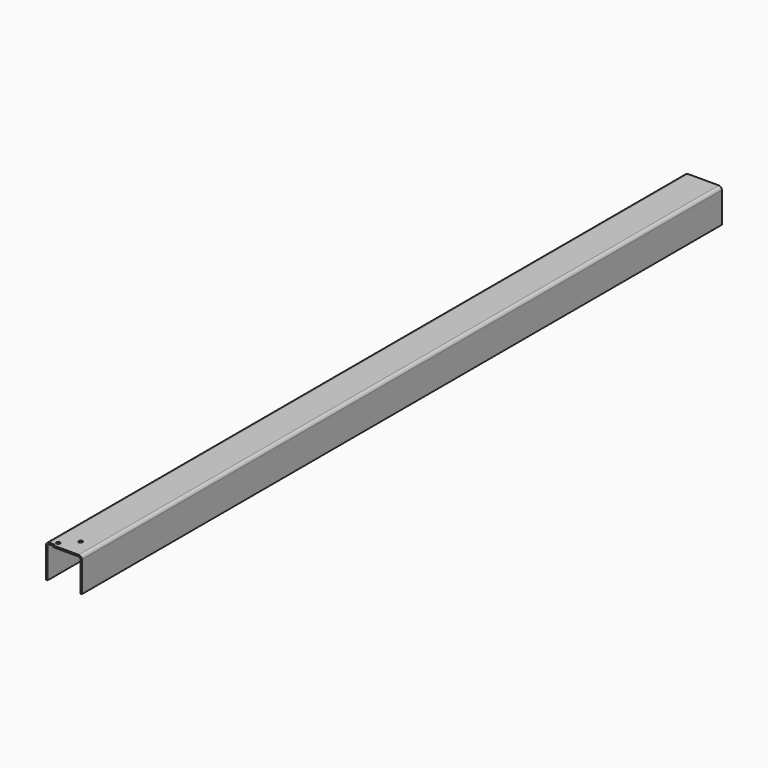
from build123d import *

# Parameters (mm, degrees)
F1_DEPTH = 1996
F3_W     = 4
F3_H     = 87
F4_DEPTH = 21.409
F6_DEPTH = 4.001


with BuildPart() as f1:
    # F0 (on Front) → F1 (new body)
    with BuildSketch(Plane.XZ):
        with BuildLine():
            Line((-46.25, 34), (-46.25, -42))
            Line((-46.25, -42), (-42.25, -42))
            Line((-42.25, -42), (-42.25, 34))
            ThreePointArc((-42.25, 34), (-41.0784271247, 36.8284271247), (-38.25, 38))
            Line((-38.25, 38), (38.25, 38))
            ThreePointArc((38.25, 38), (41.0784271247, 36.8284271247), (42.25, 34))
            Line((42.25, 34), (42.25, -42))
            Line((42.25, -42), (46.25, -42))
            Line((46.25, -42), (46.25, 34))
            ThreePointArc((46.25, 34), (43.9068542495, 39.6568542495), (38.25, 42))
            Line((38.25, 42), (-38.25, 42))
            ThreePointArc((-38.25, 42), (-43.9068542495, 39.6568542495), (-46.25, 34))
        make_face()
    extrude(amount=-F1_DEPTH)

    # F3 (on face) → F4 (cut)
    with BuildSketch(Plane(origin=(-46.25, 0, 0), x_dir=(0, -1, 0), z_dir=(-1, 0, 0))):
        with Locations((-2, 0.3707238951)):
            Rectangle(F3_W, F3_H)
    extrude(amount=-F4_DEPTH, mode=Mode.SUBTRACT)

    # F5 (on face) → F6 (cut, through all)
    with BuildSketch(Plane(origin=(0, 0, 38), x_dir=(1, 0, 0), z_dir=(0, 0, -1))):
        with BuildLine():
            ThreePointArc((-19.7495876579, -14.5), (-21.0676071426, -11.3180194847), (-24.2495876579, -10))
            ThreePointArc((-24.2495876579, -10), (-28.7495876579, -14.5), (-24.2495876579, -19))
            ThreePointArc((-24.2495876579, -19), (-21.0676071426, -17.6819805153), (-19.7495876579, -14.5))
        make_face()
        with BuildLine():
            ThreePointArc((11.2504123421, -45.5), (9.9323928574, -42.3180194847), (6.7504123421, -41))
            ThreePointArc((6.7504123421, -41), (3.5684318267, -42.3180194847), (2.2504123421, -45.5))
            ThreePointArc((2.2504123421, -45.5), (6.7504123421, -50), (11.2504123421, -45.5))
        make_face()
    extrude(amount=-F6_DEPTH, mode=Mode.SUBTRACT)


solid = f1.part
